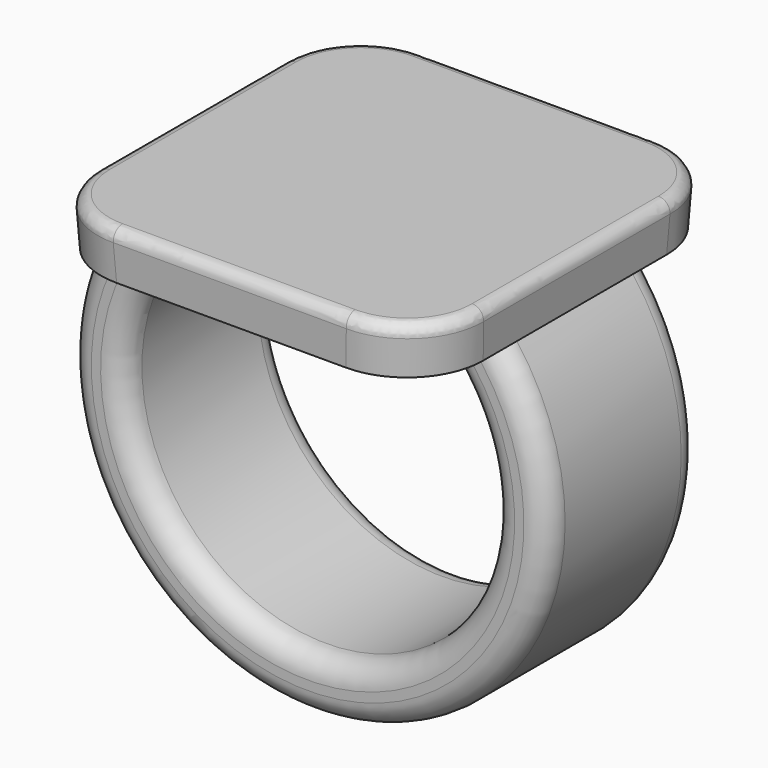
from build123d import *

# Parameters (mm, degrees)
F0_W     = 25.4
F0_H     = 25.4
F1_DEPTH = 3.175
F1_TAPER = -3
F3_W     = 5.08
F3_H     = 12.7
F5_R     = 5.08
F6_R     = 1.524
F7_R     = 0.762


with BuildPart() as f1:
    # F0 (on Top) → F1 (new body)
    with BuildSketch(Plane.XY):
        Rectangle(F0_W, F0_H)
    extrude(amount=F1_DEPTH, taper=F1_TAPER)

    # F4: sweep along a path in F2
    with BuildLine(Plane.XZ) as f4_path:
        ThreePointArc((-10.16, 0), (0, -23.5582897328), (10.16, 0))
    # F3 (on face) → F4 (sweep)
    with BuildSketch(Plane(origin=(0, 0, 0), x_dir=(1, 0, 0), z_dir=(0, 0, -1))):
        with Locations((-10.16, 0)):
            Rectangle(F3_W, F3_H)
    sweep(path=f4_path.line)

    # F5
    f5_edges = [f1.edges().sort_by_distance(p)[0] for p in [
        (12.783197, -12.783197, 1.5875),
        (-12.783197, -12.783197, 1.5875),
        (-12.783197, 12.783197, 1.5875),
        (12.783197, 12.783197, 1.5875),
    ]]
    fillet(f5_edges, radius=F5_R)

    # F6
    f6_edges = [f1.edges().sort_by_distance(p)[0] for p in [
        (-1.743325, -6.35, -21.711017),
        (-1.743325, 6.35, -21.711017),
        (0, 6.35, -25.501344),
        (0, -6.35, -25.501344),
    ]]
    fillet(f6_edges, radius=F6_R)

    # F7
    f7_edges = [f1.edges().sort_by_distance(p)[0] for p in [
        (12.866395, 0, 3.175),
        (11.381378, -11.381378, 3.175),
        (11.381378, 11.381378, 3.175),
        (0, -12.866395, 3.175),
        (0, 12.866395, 3.175),
        (-11.381378, -11.381378, 3.175),
        (-11.381378, 11.381378, 3.175),
        (-12.866395, 0, 3.175),
    ]]
    fillet(f7_edges, radius=F7_R)


solid = f1.part
